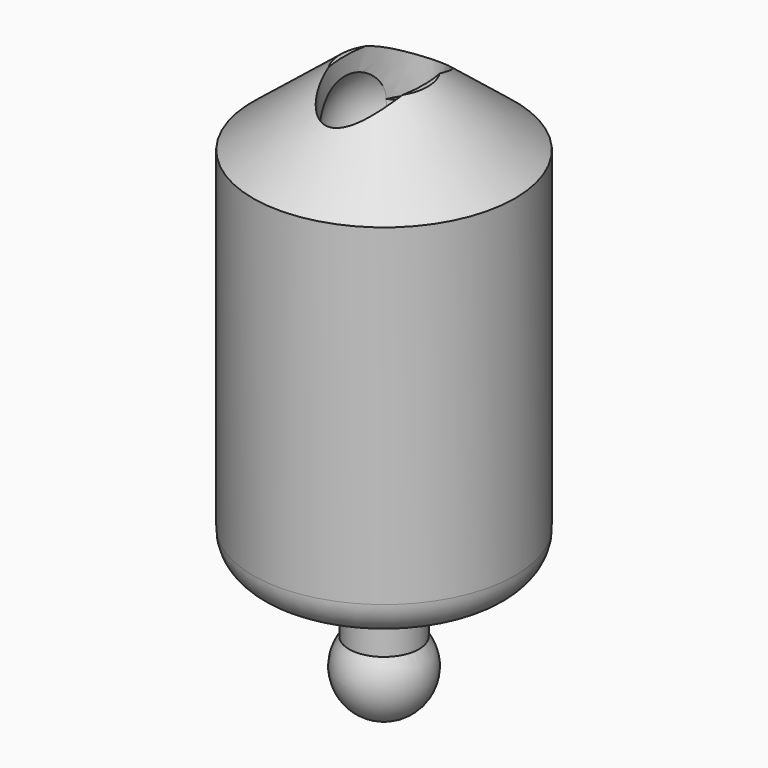
from build123d import *

# Parameters (mm, degrees)
F0_R     = 7.5
F1_DEPTH = 25
F2_R     = 2
F3_DEPTH = 5
F7_DEPTH = 3
F11_R    = 2


# Not quite as in the source:
# - a fillet or chamfer that OpenCascade refuses, or shapes differently, is made with other operations: its cross-section is extruded or revolved along the edge and cut away or added


with BuildPart() as f1:
    # F0 (on Top) → F1 (new body)
    with BuildSketch(Plane.XY):
        Circle(F0_R)
    extrude(amount=F1_DEPTH)

    # F2 (on face) → F3 (join)
    with BuildSketch(Plane(origin=(0, 0, 0), x_dir=(1, 0, 0), z_dir=(0, 0, -1))):
        Circle(F2_R)
    extrude(amount=F3_DEPTH)

    # F4 (on face) → F5 (revolve)
    with BuildSketch(Plane(origin=(0, 0, -5), x_dir=(1, 0, 0), z_dir=(0, 0, -1))):
        with BuildLine():
            Line((0, 2), (0, 2.5))
            ThreePointArc((0, 2.5), (-2.5, 0), (0, -2.5))
            Line((0, -2.5), (0, -2))
            ThreePointArc((0, -2), (-2, 0), (0, 2))
        make_face()
        with BuildLine():
            Line((0, -2), (0, 2))
            ThreePointArc((0, 2), (-2, 0), (0, -2))
        make_face()
    revolve(axis=Axis((0, 0, -5), (0, 1, 0)))

    # F6 (on face) → F7 (cut)
    with BuildSketch(Plane.XY.offset(25)):
        with BuildLine():
            add(Edge.make_bspline(
                [(0, 4), (-3.897114317, 4), (-1.9485571585, -2), (0, -8), (1.9485571585, -2), (3.897114317, 4), (0, 4)],
                knots=[0, 0, 0, 2.0943951024, 2.0943951024, 4.1887902048, 4.1887902048, 6.2831853072, 6.2831853072, 6.2831853072], degree=2, weights=[1, 0.5, 1, 0.5, 1, 0.5, 1]))
        make_face()
    extrude(amount=-F7_DEPTH, mode=Mode.SUBTRACT)

    # F8 (on face) → F9 (revolve, cut)
    with BuildSketch(Plane.XY.offset(22)):
        with BuildLine():
            ThreePointArc((1.8, -2.4), (2.683281573, -1.3416407865), (3, 0))
            ThreePointArc((3, 0), (2.683281573, 1.3416407865), (1.8, 2.4))
            add(Edge.make_bspline(
                [(1.8, -2.4), (1.8810311774, -2.2079260981), (1.9485571585, -2), (2.6913429511, 0.2871870789), (1.8, 2.4)],
                knots=[4.0484923357, 4.0484923357, 4.0484923357, 4.1887902048, 4.1887902048, 5.3448576064, 5.3448576064, 5.3448576064], degree=2, weights=[0.9375, 0.9665063509, 1, 0.7240092377, 0.7527020789]))
        make_face()
        with BuildLine():
            Line((0, -3), (0, 3))
            ThreePointArc((0, 3), (-0.9486832981, 2.8460498942), (-1.8, 2.4))
            add(Edge.make_bspline(
                [(-1.8, 2.4), (-2.6913429511, 0.2871870789), (-1.9485571585, -2), (-1.8810311774, -2.2079260981), (-1.8, -2.4)],
                knots=[0.9383277008, 0.9383277008, 0.9383277008, 2.0943951024, 2.0943951024, 2.2346929715, 2.2346929715, 2.2346929715], degree=2, weights=[0.7527020789, 0.7240092377, 1, 0.9665063509, 0.9375]))
            ThreePointArc((-1.8, -2.4), (-0.9486832981, -2.8460498942), (0, -3))
        make_face()
    revolve(axis=Axis((0, 0, 22), (0, -1, 0)), mode=Mode.SUBTRACT)

    # F10: chamfer of 5 x 4 on 1 edges, made by hand

    # F10_s1 → F10_t2 (revolve, cut)
    with BuildSketch(Plane.XZ):
        Polygon((7.5, 21), (2.5, 25), (7.5, 25), align=None)
    revolve(axis=Axis((0, 0, 25), (0, 0, 1)), mode=Mode.SUBTRACT)

    # F11
    f11_edges = [f1.edges().sort_by_distance(p)[0] for p in [
        (-7.5, 0, 0),
    ]]
    fillet(f11_edges, radius=F11_R)


solid = f1.part
